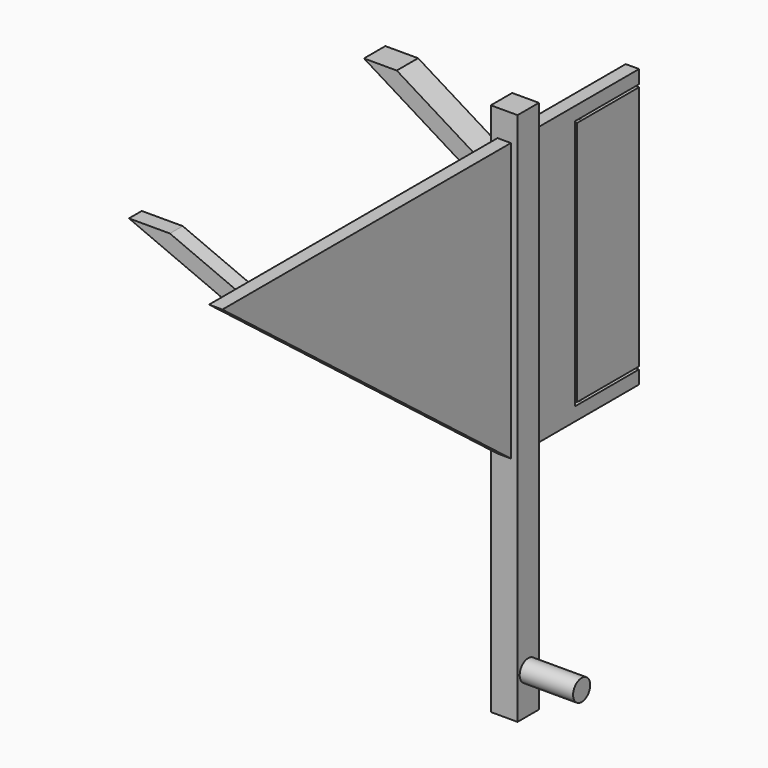
from build123d import *

# Parameters (mm, degrees)
F0_W      = 10
F0_H      = 200
F1_DEPTH  = 10
F3_DEPTH  = 135
F5_DEPTH  = 7.501
F6_W      = 6
F6_H      = 6
F6_H_2    = 7.259
F6_H_3    = 2
F7_DEPTH  = 50
F9_DEPTH  = 6
F10_W     = 5
F10_H     = 10
F10_H_2   = 9.253
F11_DEPTH = 47.5
F13_DEPTH = 10
F15_DEPTH = 20
F17_DEPTH = 50
F19_DEPTH = 5
F21_DEPTH = 92
F23_DEPTH = 94


# Not quite as in the source:
# - a feature names something its author has since deleted; it is built from what else it names


with BuildPart() as f1:
    # F0 (on Front) → F1 (new body)
    with BuildSketch(Plane.XZ):
        Rectangle(F0_W, F0_H)
    extrude(amount=F1_DEPTH)

    # F2 (on face) → F3 (join)
    with BuildSketch(Plane.XZ.offset(10)):
        Polygon((2.5, 90), (0, 90), (-2.5, 90), (-2.5, -14), (0, -14), (2.5, -14), align=None)
    extrude(amount=F3_DEPTH)

    # F4 (on face) → F5 (cut, through all)
    with BuildSketch(Plane.YZ.offset(2.5)):
        Polygon((-10, -14), (-145, 90), (-145, -14), align=None)
    extrude(amount=-F5_DEPTH, mode=Mode.SUBTRACT)

    # F6 (on face) → F7 (join)
    with BuildSketch(Plane(origin=(-2.5, 0, 0), x_dir=(0, -1, 0), z_dir=(-1, 0, 0))):
        with Locations((117, 87)):
            Rectangle(F6_W, F6_H)
        with Locations((117, 73.741)):
            Rectangle(F6_W, F6_H)
        with Locations((117, 80.3705)):
            Rectangle(F6_W, F6_H_2)
        with Locations((117, 91)):
            Rectangle(F6_W, F6_H_3)
    extrude(amount=F7_DEPTH)

    # F8 (on face) → F9 (cut, through all)
    with BuildSketch(Plane.XZ.offset(120)):
        Polygon((-52.5, 70.741), (-2.5, 70.741), (-52.5, 92), align=None)
        Polygon((-37.1657494443, 92), (-2.5, 77.2608166513), (-2.5, 90), (-2.5, 92), align=None)
    extrude(amount=-F9_DEPTH, mode=Mode.SUBTRACT)

    # F10 (on face) → F11 (join)
    with BuildSketch(Plane(origin=(-5, 0, 0), x_dir=(0, -1, 0), z_dir=(-1, 0, 0))):
        with Locations((7.5, 75.747)):
            Rectangle(F10_W, F10_H)
        with Locations((2.5, 75.747)):
            Rectangle(F10_W, F10_H)
        with Locations((2.5, 85.3735)):
            Rectangle(F10_W, F10_H_2)
        with Locations((7.5, 85.3735)):
            Rectangle(F10_W, F10_H_2)
        with Locations((7.5, 95)):
            Rectangle(F10_W, F10_H)
        with Locations((2.5, 95)):
            Rectangle(F10_W, F10_H)
    extrude(amount=F11_DEPTH)

    # F12 (on face) → F13 (cut, through all)
    with BuildSketch(Plane.XZ.offset(10)):
        Polygon((-5, 70.747), (-52.5, 100), (-52.5, 70.747), align=None)
        Polygon((-5, 100), (-40.2273908257, 100), (-5, 78.3051186563), align=None)
    extrude(amount=-F13_DEPTH, mode=Mode.SUBTRACT)

    # F14 (on face) → F15 (join)
    with BuildSketch(Plane.YZ.offset(5)):
        with BuildLine():
            ThreePointArc((-1, -85), (-7.8284271247, -82.1715728753), (-5, -89))
            ThreePointArc((-5, -89), (-2.1715728753, -87.8284271247), (-1, -85))
        make_face()
    extrude(amount=F15_DEPTH)

    # F16 (on face) → F17 (join)
    with BuildSketch(Plane(origin=(0, 0, 0), x_dir=(-1, 0, 0), z_dir=(0, 1, 0))):
        Polygon((2.5, 90), (0, 90), (-2.5, 90), (-2.5, -14), (2.5, -14), align=None)
    extrude(amount=F17_DEPTH)

    # F18 (on face) → F19 (cut, through all)
    with BuildSketch(Plane.YZ.offset(2.5)):
        Polygon((50, 84), (50, 85), (20, 85), (20, -9), (50, -9), (50, -8), (21, -8), (21, 84), align=None)
    extrude(amount=-F19_DEPTH, mode=Mode.SUBTRACT)

    # F20 (on face) → F21 (cut, through all)
    with BuildSketch(Plane.XY.offset(84)):
        with BuildLine():
            ThreePointArc((0, 22.5), (1.0606601718, 22.9393398282), (1.5, 24))
            ThreePointArc((1.5, 24), (-1.0606601718, 25.0606601718), (0, 22.5))
        make_face()
    extrude(amount=-F21_DEPTH, mode=Mode.SUBTRACT)


with BuildPart() as f23:
    # F22 (on face) → F23 (new body, through all)
    with BuildSketch(Plane(origin=(0, 0, 85), x_dir=(1, 0, 0), z_dir=(0, 0, -1))):
        with BuildLine():
            ThreePointArc((1.5, -24), (1.0606601718, -22.9393398282), (0, -22.5))
            Line((0, -22.5), (0, -24))
            Line((0, -24), (0, -25.5))
            ThreePointArc((0, -25.5), (1.0606601718, -25.0606601718), (1.5, -24))
        make_face()
        with BuildLine():
            Line((0, -24), (0, -22.5))
            ThreePointArc((0, -22.5), (-1.5, -24), (0, -25.5))
            Line((0, -25.5), (0, -24))
        make_face()
    extrude(amount=F23_DEPTH)


solid = Compound([f1.part, f23.part])
